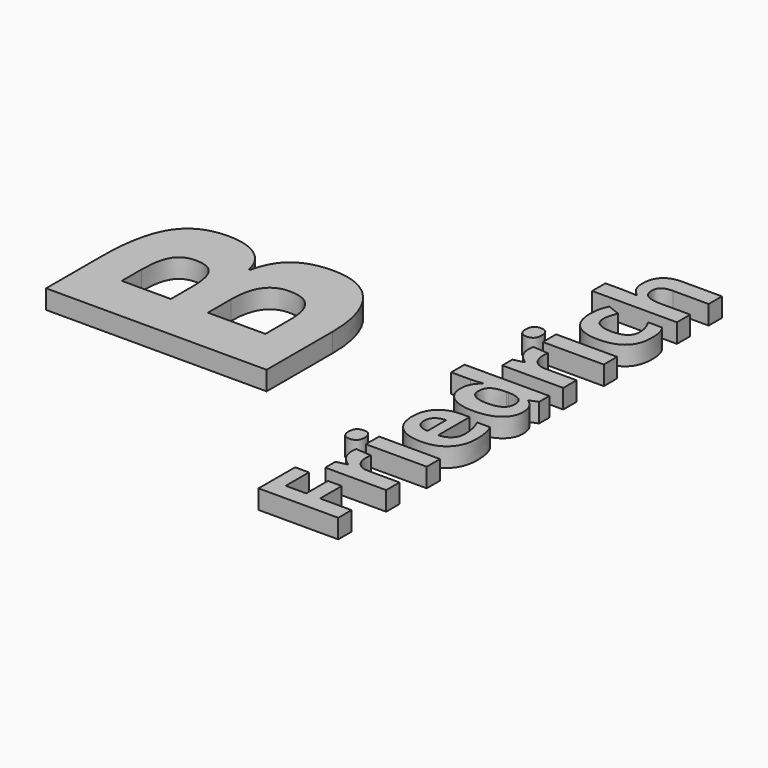
from build123d import *

# Parameters (mm, degrees)
F0_TEXT_SIZE   = 64.8916396261
F0_TEXT_SIZE_2 = 23.4460130341
F1_DEPTH       = 4


# Not quite as in the source:
# - Text() gives the source's letters only with a copy of the font that has no kerning and outlines rounded to 1/6400 em; it was checked with that copy


with BuildPart() as f1:
    # F0 (on Top) → F1 (new body)
    with BuildSketch(Plane.XY):
        with Locations(Location((0, -22.1949686158), (0, 0, 90))):
            Text('B', F0_TEXT_SIZE, font='Open Sans', font_style=FontStyle.BOLD, text_align=(TextAlign.LEFT, TextAlign.BOTTOM))
        with Locations(Location((42.0279229586, -52.1911904216), (0, 0, 90))):
            Text('Friedrich', F0_TEXT_SIZE_2, font='Open Sans', font_style=FontStyle.BOLD, text_align=(TextAlign.LEFT, TextAlign.BOTTOM))
    extrude(amount=-F1_DEPTH)


solid = f1.part
